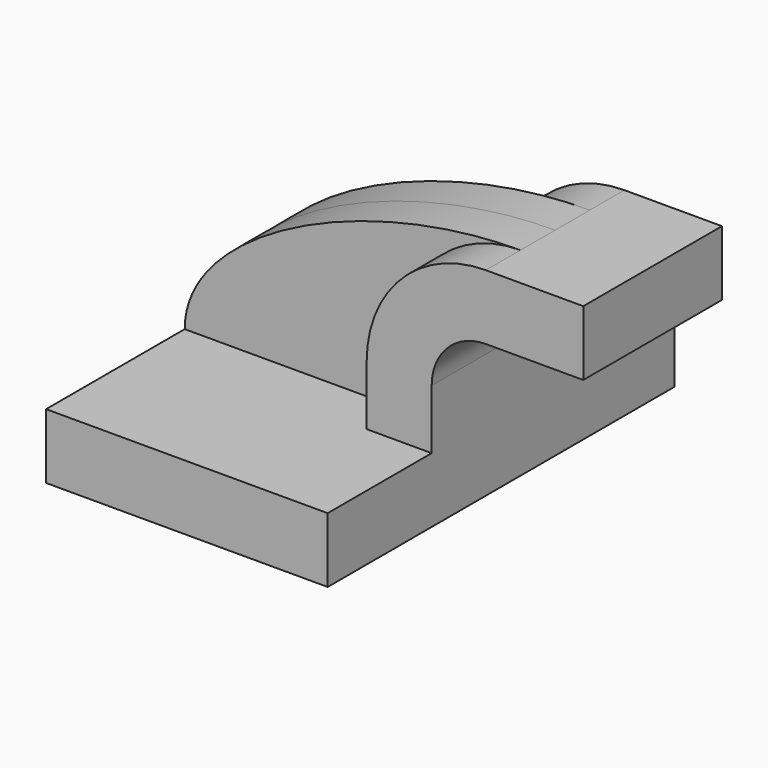
from build123d import *

# Parameters (mm, degrees)
F1_DEPTH = 63.5
F0_W     = 25.4
F0_H     = 19.05
F2_DEPTH = 25.4
F3_DEPTH = 12.7


with BuildPart() as f1:
    # F0 (on Front) → F1 (new body, symmetric)
    with BuildSketch(Plane.XZ):
        Polygon((41.275, -9.525), (41.275, 9.525), (22.225, 9.525), (-41.275, 9.525), (-41.275, -9.525), align=None)
    extrude(amount=F1_DEPTH, both=True)

    # F0 (on Front) → F2 (join, symmetric)
    with BuildSketch(Plane.XZ):
        with BuildLine():
            Line((22.225, 9.525), (41.275, 9.525))
            Line((41.275, 9.525), (41.275, 26.9875))
            ThreePointArc((41.275, 26.9875), (45.9246798487, 38.2128201513), (57.15, 42.8625))
            Line((57.15, 42.8625), (60.325, 42.8625))
            Line((60.325, 42.8625), (60.325, 61.9125))
            Line((60.325, 61.9125), (57.15, 61.9125))
            ThreePointArc((57.15, 61.9125), (32.4542956671, 51.6832043329), (22.225, 26.9875))
            Line((22.225, 26.9875), (22.225, 9.525))
        make_face()
        with Locations((73.025, 52.3875)):
            Rectangle(F0_W, F0_H)
    extrude(amount=F2_DEPTH, both=True)

    # F0 (on Front) → F3 (join, symmetric)
    with BuildSketch(Plane.XZ):
        with BuildLine():
            Line((-41.275, 9.525), (22.225, 9.525))
            Line((22.225, 9.525), (22.225, 26.9875))
            ThreePointArc((22.225, 26.9875), (32.4542956671, 51.6832043329), (57.15, 61.9125))
            add(Edge.make_bspline(
                [(-41.275, 9.525), (-41.275, 36.84458516), (10.5578337313, 61.9125), (57.15, 61.9125)],
                knots=[0, 0, 0, 0, 111.4985685166, 111.4985685166, 111.4985685166, 111.4985685166], degree=3))
        make_face()
    extrude(amount=F3_DEPTH, both=True)


solid = f1.part
